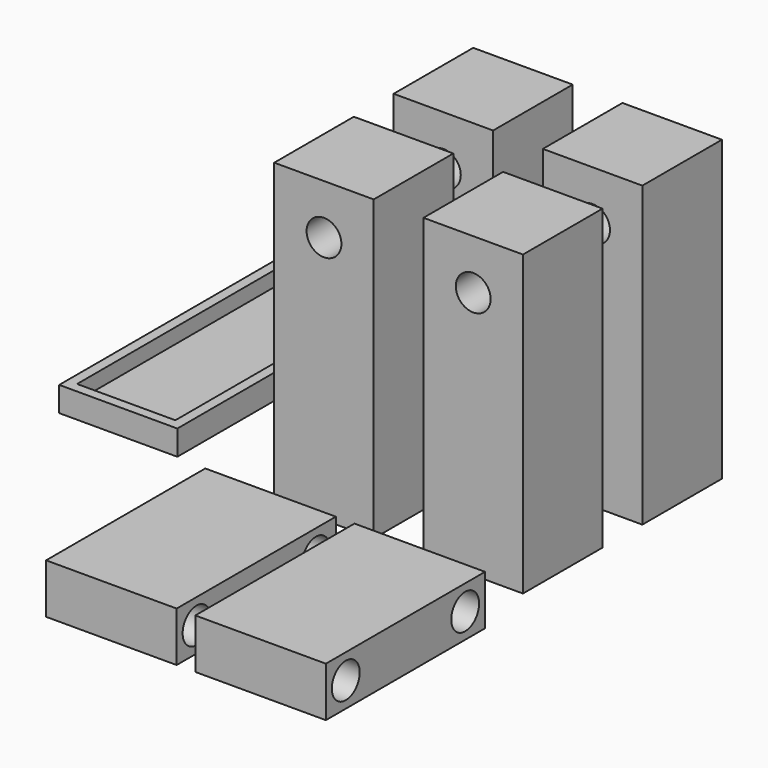
from build123d import *

# Parameters (mm, degrees)
F0_W      = 30.1625
F0_H      = 69.85
F1_DEPTH  = 6.35
F2_T      = -2.54
F3_W      = 25.4
F3_H      = 76.2
F3_R      = 4.445
F4_DEPTH  = 25.4
F9_W      = 50.8
F9_H      = 12.7
F9_R      = 4.445
F10_DEPTH = 33.3375


with BuildPart() as f1:
    # F0 (on Top) → F1 (new body)
    with BuildSketch(Plane.XY):
        with Locations((-37.8125467181, 37.9975575052)):
            Rectangle(F0_W, F0_H)
    extrude(amount=F1_DEPTH)

    # F2
    f2_openings = [f1.faces().sort_by_distance(p)[0] for p in [
        (-37.812547, 37.997558, 6.35),
    ]]
    offset(amount=F2_T, openings=f2_openings)


with BuildPart() as f4:
    # F3 (on Front) → F4 (new body)
    with BuildSketch(Plane.XZ):
        with Locations((17.1653133214, 38.1)):
            Rectangle(F3_W, F3_H)
        with Locations((17.1653133214, 63.5)):
            Circle(F3_R, mode=Mode.SUBTRACT)
    extrude(amount=F4_DEPTH)


with BuildPart() as f4_1:
    # F5: moved
    add(f4.part.moved(Location((0, 25.4, 0))))


with BuildPart() as f6_1:
    # F6: copy of F4
    add(f4_1.part.moved(Location((38.1, 0, 0))))


with BuildPart() as f7_1:
    # F7: copy of F4
    add(f4_1.part.moved(Location((0, 38.1, 0))))


with BuildPart() as f8_1:
    # F8: copy of F4
    add(f4_1.part.moved(Location((38.1, 38.1, 0))))


with BuildPart() as f10:
    # F9 (on Right) → F10 (new body)
    with BuildSketch(Plane.YZ):
        with Locations((-41.8334656119, 6.35)):
            Rectangle(F9_W, F9_H)
        with Locations((-60.8834656119, 6.35)):
            Circle(F9_R, mode=Mode.SUBTRACT)
        with Locations((-22.7834656119, 6.35)):
            Circle(F9_R, mode=Mode.SUBTRACT)
    extrude(amount=F10_DEPTH)


with BuildPart() as f11_1:
    # F11: copy of F10
    add(f10.part.moved(Location((38.1, 0, 0))))


solid = Compound([f1.part, f4_1.part, f6_1.part, f7_1.part, f8_1.part, f10.part, f11_1.part])
